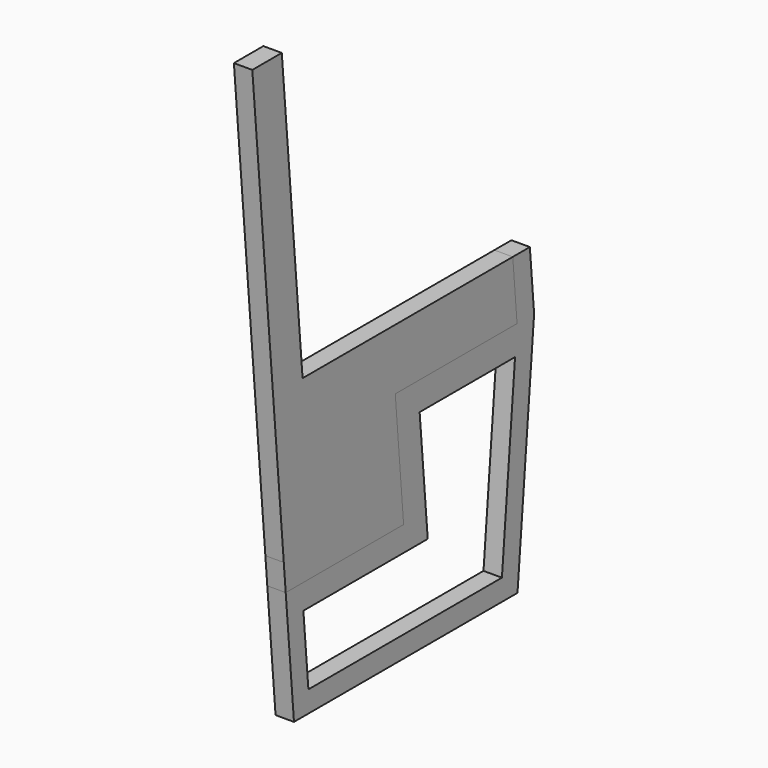
from build123d import *

# Parameters (mm, degrees)
F1_DEPTH = 25.4
F2_DEPTH = 25.4


# Not quite as in the source:
# - a feature names something its author has since deleted; it is built from what else it names


with BuildPart() as f1:
    # F0 (on Right) → F1 (new body)
    with BuildSketch(Plane.YZ):
        Polygon((-2.8831724243, 200.7012711329), (0.4370540533, 162.7509088374), (203.6370540533, 162.7509088374), (189.2476409256, 327.2226534924), (399.1505950094, 327.2226534924), (391.8048532493, 411.1848660134), (29.5018991655, 411.1848660134), (-6.3205984573, 820.6378874572), (-57.1205984573, 820.6378874572), (-21.1470656382, 409.4585258199), align=None)
    extrude(amount=F1_DEPTH)


with BuildPart() as f2:
    # F0 (on Right) → F2 (new body)
    with BuildSketch(Plane.YZ):
        Polygon((0.4370540533, 162.7509088374), (14.6759135551, 0), (42.1129448534, 0), (39.5412336167, 29.3947939436), (30.8813626048, 128.3775725444), (205.7059179631, 128.3775725444), (245.2201617377, 128.3775725444), (231.2555789637, 287.9934840373), (395.7184874025, 287.9934840373), (399.1505950094, 327.2226534924), (189.2476409256, 327.2226534924), (203.6370540533, 162.7509088374), align=None)
        Polygon((391.8048532493, 411.1848660134), (399.1505950094, 327.2226534924), (428.5714484425, 327.2258416546), (421.2259856104, 411.1848660134), align=None)
        Polygon((428.5714484425, 327.2258416546), (399.1505950094, 327.2226534924), (395.7184874025, 287.9934840373), (373.0940336167, 29.3947939436), (370.5223223799, 0), (399.942896885, 0), align=None)
        Polygon((39.5412336167, 29.3947939436), (42.1129448534, 0), (216.9375002117, 0), (256.4517439863, 0), (253.8800327496, 29.3947939436), align=None)
        Polygon((253.8800327496, 29.3947939436), (256.4517439863, 0), (370.5223223799, 0), (373.0940336167, 29.3947939436), align=None)
    extrude(amount=F2_DEPTH)


solid = Compound([f1.part, f2.part])
